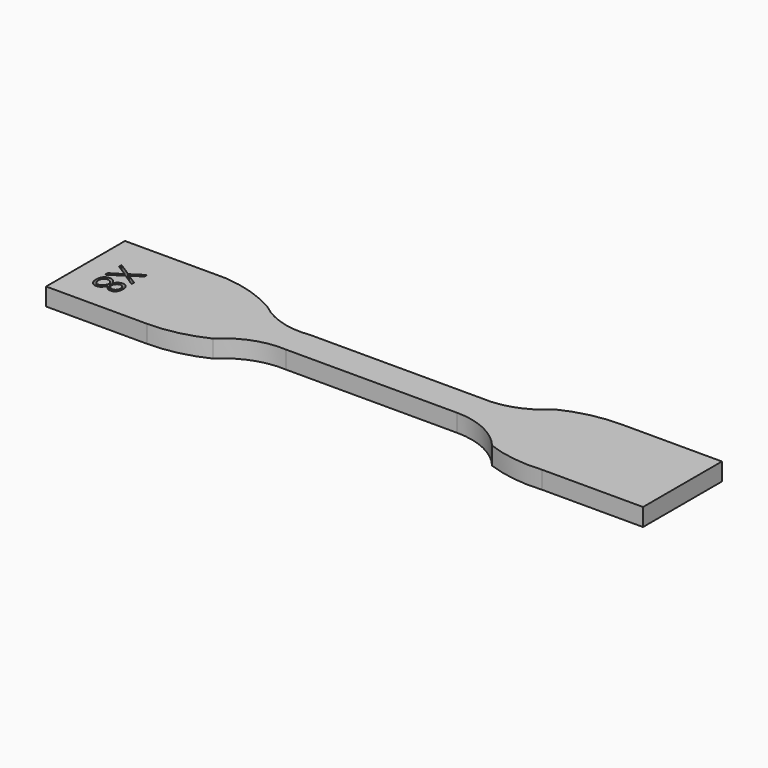
from build123d import *

# Parameters (mm, degrees)
F1_DEPTH     = 3.4
F2_TEXT_SIZE = 7.0564552314
F3_DEPTH     = 1


# Not quite as in the source:
# - Text() gives the source's letters only with a copy of the font that has no kerning and outlines rounded to 1/6400 em; it was checked with that copy


with BuildPart() as f1:
    # F0 (on Top) → F1 (new body)
    with BuildSketch(Plane.XY):
        with BuildLine():
            Line((-14.4320548165, 19.7811394548), (-33.8720548165, 19.7811394548))
            Line((-33.8720548165, 19.7811394548), (-33.8720548165, 0.7811394548))
            Line((-33.8720548165, 0.7811394548), (-14.4320548165, 0.7811394548))
            ThreePointArc((-14.4320548165, 0.7811394548), (-8.9053122052, 1.3996892086), (-3.6520548165, 3.2247301661))
            ThreePointArc((-3.6520548165, 3.2247301661), (1.3014698263, 6.4128780055), (7.1279451835, 7.2811394548))
            Line((7.1279451835, 7.2811394548), (40.1279451835, 7.2811394548))
            ThreePointArc((40.1279451835, 7.2811394548), (46.0837574042, 5.9511158081), (50.9079451835, 2.2137538538))
            ThreePointArc((50.9079451835, 2.2137538538), (56.2191047011, 0.9041953221), (61.6879451835, 0.7811394548))
            Line((61.6879451835, 0.7811394548), (81.1279451835, 0.7811394548))
            Line((81.1279451835, 0.7811394548), (81.1279451835, 19.7811394548))
            Line((81.1279451835, 19.7811394548), (61.6879451835, 19.7811394548))
            ThreePointArc((61.6879451835, 19.7811394548), (56.1612025723, 19.162589701), (50.9079451835, 17.3375487435))
            ThreePointArc((50.9079451835, 17.3375487435), (45.9544205407, 14.1494009041), (40.1279451835, 13.2811394548))
            Line((40.1279451835, 13.2811394548), (7.1279451835, 13.2811394548))
            ThreePointArc((7.1279451835, 13.2811394548), (1.4167452884, 13.6925537245), (-3.6520548165, 16.3560723447))
            ThreePointArc((-3.6520548165, 16.3560723447), (-8.8458057958, 18.686276846), (-14.4320548165, 19.7811394548))
        make_face()
    extrude(amount=F1_DEPTH)

    # F2 (on face) → F3 (cut)
    with BuildSketch(Plane.XY.offset(3.4)):
        with Locations(Location((-29.3720550835, 13.353464842), (0, 0, -90))):
            Text('X8', F2_TEXT_SIZE, font='Open Sans', text_align=(TextAlign.LEFT, TextAlign.BOTTOM))
    extrude(amount=-F3_DEPTH, mode=Mode.SUBTRACT)


solid = f1.part
